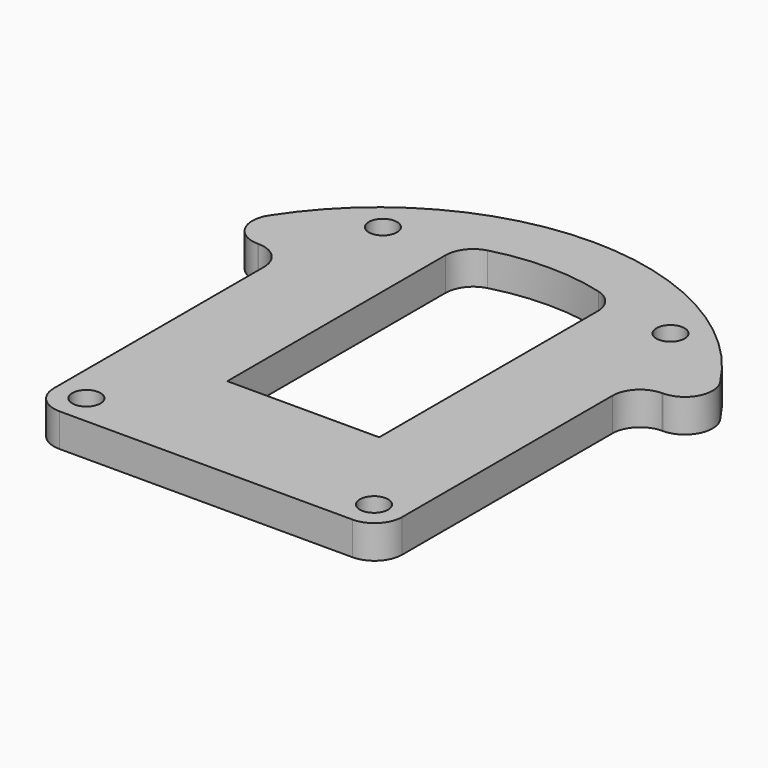
from build123d import *

# Parameters (mm, degrees)
F0_R     = 2.55
F0_W     = 27.4615384615
F0_H     = 34
F1_DEPTH = 6
F2_R     = 2.55
F3_DEPTH = 6
F5_DEPTH = 6.001
F6_R     = 5


with BuildPart() as f1:
    # F0 (on Top) → F1 (new body)
    with BuildSketch(Plane.XY):
        with BuildLine():
            Line((26.5, 39), (-26.5, 39))
            ThreePointArc((-26.5, 39), (-30.0355339059, 37.5355339059), (-31.5, 34))
            Line((-31.5, 34), (-31.5, -34))
            ThreePointArc((-31.5, -34), (-30.0355339059, -37.5355339059), (-26.5, -39))
            Line((-26.5, -39), (26.5, -39))
            ThreePointArc((26.5, -39), (30.0355339059, -37.5355339059), (31.5, -34))
            Line((31.5, -34), (31.5, 34))
            ThreePointArc((31.5, 34), (30.0355339059, 37.5355339059), (26.5, 39))
        make_face()
        with Locations((-26, -33.5)):
            Circle(F0_R, mode=Mode.SUBTRACT)
        with Locations((26, -33.5)):
            Circle(F0_R, mode=Mode.SUBTRACT)
        Rectangle(F0_W, F0_H, mode=Mode.SUBTRACT)
        with Locations((-26, 33.5)):
            Circle(F0_R, mode=Mode.SUBTRACT)
        with Locations((26, 33.5)):
            Circle(F0_R, mode=Mode.SUBTRACT)
    extrude(amount=F1_DEPTH)

    # F2 (on Top) → F3 (join, through all)
    with BuildSketch(Plane.XY):
        with BuildLine():
            Line((-44.8330235429, 18.5), (44.8330235429, 18.5))
            ThreePointArc((44.8330235429, 18.5), (0, 48.5), (-44.8330235429, 18.5))
        make_face()
        with Locations((-26, 33.5)):
            Circle(F2_R, mode=Mode.SUBTRACT)
        with Locations((26, 33.5)):
            Circle(F2_R, mode=Mode.SUBTRACT)
    extrude(amount=F3_DEPTH)

    # F4 (on Top) → F5 (cut, through all)
    with BuildSketch(Plane.XY):
        with BuildLine():
            Line((13.7307692308, 17), (13.7307692308, 35.96826346))
            ThreePointArc((13.7307692308, 35.96826346), (0, 38.5), (-13.7307692308, 35.96826346))
            Line((-13.7307692308, 35.96826346), (-13.7307692308, 17))
            Line((-13.7307692308, 17), (13.7307692308, 17))
        make_face()
    extrude(amount=F5_DEPTH, mode=Mode.SUBTRACT)

    # F6
    f6_edges = [f1.edges().sort_by_distance(p)[0] for p in [
        (44.833024, 18.5, 3),
        (-31.5, 18.5, 3),
        (31.5, 18.5, 3),
        (13.730769, 35.968263, 3),
        (-13.730769, 35.968263, 3),
        (-44.833024, 18.5, 3),
    ]]
    fillet(f6_edges, radius=F6_R)


solid = f1.part
